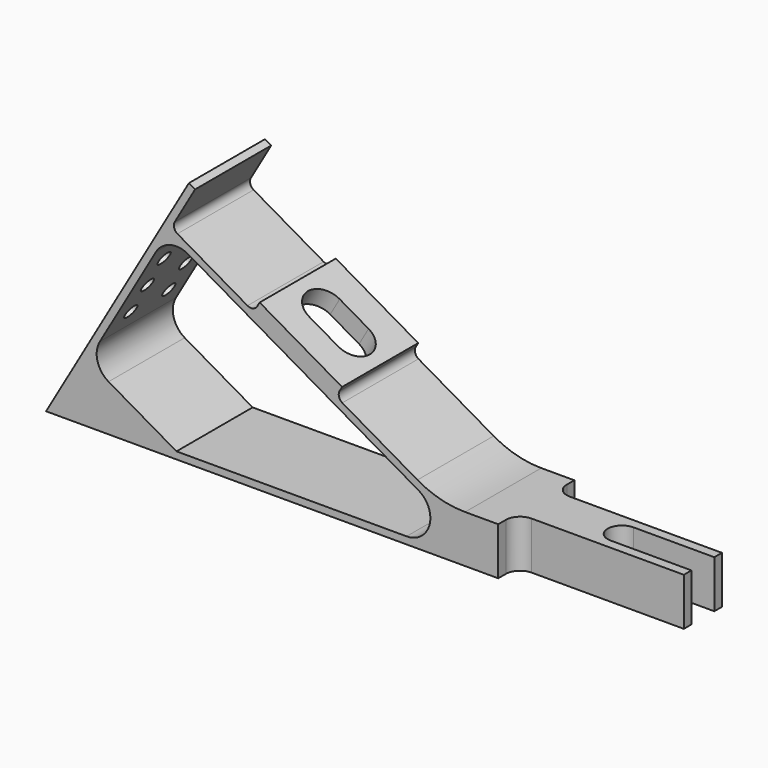
from build123d import *

# Parameters (mm, degrees)
F1_DEPTH      = 10
F3_DEPTH      = 20.001
F3_DEPTH_BACK = 197
F4_R          = 1.5
F5_DEPTH      = 1.5
F4_R_2        = 4.25
F6_DEPTH      = 112.584302492
F4_R_3        = 5.5
F7_DEPTH      = 2
F8_W          = 17
F8_H          = 6
F9_DEPTH      = 10.001
F10_W         = 7
F10_H         = 8
F11_DEPTH     = 4


# Not quite as in the source:
# - an extrude ends at something that could not be found from the text; its depth is read off the source's solid


with BuildPart() as f1:
    # F0 (on Front) → F1 (new body, symmetric)
    with BuildSketch(Plane.XZ):
        with BuildLine():
            Line((30, 51.9615242271), (0, 0))
            Line((0, 0), (130, 0))
            Line((130, 0), (130, 10))
            Line((130, 10), (88.0384757729, 10))
            ThreePointArc((88.0384757729, 10), (82.8620948709, 10.6814834742), (78.0384757729, 12.6794919243))
            Line((78.0384757729, 12.6794919243), (62.2390923627, 21.8012701892))
            ThreePointArc((62.2390923627, 21.8012701892), (61.5402036233, 22.7120797272), (61.6900542571, 23.8503082949))
            Line((61.6900542571, 23.8503082949), (62.1900542571, 24.7163336987))
            Line((62.1900542571, 24.7163336987), (44.8695461814, 34.7163336987))
            Line((44.8695461814, 34.7163336987), (44.3695461814, 33.8503082949))
            ThreePointArc((44.3695461814, 33.8503082949), (43.4587366433, 33.1514195555), (42.3205080757, 33.3012701892))
            Line((42.3205080757, 33.3012701892), (27.5980762114, 41.8012701892))
            ThreePointArc((27.5980762114, 41.8012701892), (26.8991874719, 42.7120797272), (27.0490381057, 43.8503082949))
            Line((27.0490381057, 43.8503082949), (31.2990381057, 51.2115242271))
            Line((31.2990381057, 51.2115242271), (30, 51.9615242271))
        make_face()
        with BuildLine():
            ThreePointArc((23.0490381057, 36.9221050646), (26.0850698991, 39.2517341961), (29.8791651246, 38.7522320835))
            Line((29.8791651246, 38.7522320835), (78.2416697508, 10.8301270189))
            ThreePointArc((78.2416697508, 10.8301270189), (80.5712988822, 5.2059047745), (75.7416697508, 1.5))
            Line((75.7416697508, 1.5), (27.4019237886, 1.5))
            Line((27.4019237886, 1.5), (13.1291651246, 9.7403810568))
            ThreePointArc((13.1291651246, 9.7403810568), (10.7995359932, 12.7764128502), (11.2990381057, 16.5705080757))
            Line((11.2990381057, 16.5705080757), (23.0490381057, 36.9221050646))
        make_face(mode=Mode.SUBTRACT)
        with BuildLine():
            Line((78.2416697508, 10.8301270189), (29.8791651246, 38.7522320835))
            ThreePointArc((29.8791651246, 38.7522320835), (26.0850698991, 39.2517341961), (23.0490381057, 36.9221050646))
            Line((23.0490381057, 36.9221050646), (11.2990381057, 16.5705080757))
            ThreePointArc((11.2990381057, 16.5705080757), (10.7995359932, 12.7764128502), (13.1291651246, 9.7403810568))
            Line((13.1291651246, 9.7403810568), (27.4019237886, 1.5))
            Line((27.4019237886, 1.5), (75.7416697508, 1.5))
            ThreePointArc((75.7416697508, 1.5), (80.5712988822, 5.2059047745), (78.2416697508, 10.8301270189))
        make_face()
    extrude(amount=F1_DEPTH, both=True)

    # F2 (on face) → F3 (cut, two sides)
    with BuildSketch(Plane.XZ.offset(10)) as f3_sk:
        with BuildLine():
            ThreePointArc((29.8791651246, 38.7522320835), (26.0850698991, 39.2517341961), (23.0490381057, 36.9221050646))
            Line((23.0490381057, 36.9221050646), (11.2990381057, 16.5705080757))
            ThreePointArc((11.2990381057, 16.5705080757), (10.7995359932, 12.7764128502), (13.1291651246, 9.7403810568))
            Line((13.1291651246, 9.7403810568), (27.4019237886, 1.5))
            Line((27.4019237886, 1.5), (75.7416697508, 1.5))
            ThreePointArc((75.7416697508, 1.5), (80.5712988822, 5.2059047745), (78.2416697508, 10.8301270189))
            Line((78.2416697508, 10.8301270189), (29.8791651246, 38.7522320835))
        make_face()
    extrude(amount=-F3_DEPTH, mode=Mode.SUBTRACT)
    extrude(f3_sk.sketch, amount=F3_DEPTH_BACK, mode=Mode.SUBTRACT)

    # F4 (on face) → F5 (cut, through all)
    with BuildSketch(Plane(origin=(0, 0, 0), x_dir=(0, -1, 0), z_dir=(-0.8660254038, 0, 0.5))):
        with Locations((-5, 25)):
            Circle(F4_R)
        with Locations((-5, 32)):
            Circle(F4_R)
        with Locations((-5, 39)):
            Circle(F4_R)
        with Locations((5, 39)):
            Circle(F4_R)
        with Locations((5, 32)):
            Circle(F4_R)
        with Locations((5, 25)):
            Circle(F4_R)
    extrude(amount=-F5_DEPTH, mode=Mode.SUBTRACT)

    # F4 (on face) → F6 (cut, through all)
    with BuildSketch(Plane(origin=(0, 0, 0), x_dir=(0, -1, 0), z_dir=(-0.8660254038, 0, 0.5))):
        with Locations((0, 10)):
            Circle(F4_R_2)
    extrude(amount=-F6_DEPTH, mode=Mode.SUBTRACT)

    # F4 (on face) → F7 (cut)
    with BuildSketch(Plane(origin=(0, 0, 0), x_dir=(0, -1, 0), z_dir=(-0.8660254038, 0, 0.5))):
        with Locations((0, 10)):
            Circle(F4_R_3)
        with Locations((0, 10)):
            Circle(F4_R_2, mode=Mode.SUBTRACT)
    extrude(amount=-F7_DEPTH, mode=Mode.SUBTRACT)

    # F8 (on face) → F9 (cut, through all)
    with BuildSketch(Plane.XY.offset(10)):
        with Locations((121.5, 0)):
            Rectangle(F8_W, F8_H)
        with BuildLine():
            ThreePointArc((113, 3), (110, 0), (113, -3))
            Line((113, -3), (113, 3))
        make_face()
        with BuildLine():
            Line((130, -10), (130, -5))
            Line((130, -5), (98, -5))
            ThreePointArc((98, -5), (95.8786796564, -5.8786796564), (95, -8))
            Line((95, -8), (95, -10))
            Line((95, -10), (130, -10))
        make_face()
        with BuildLine():
            Line((98, 5), (130, 5))
            Line((130, 5), (130, 10))
            Line((130, 10), (95, 10))
            Line((95, 10), (95, 8))
            ThreePointArc((95, 8), (95.8786796564, 5.8786796564), (98, 5))
        make_face()
    extrude(amount=-F9_DEPTH, mode=Mode.SUBTRACT)

    # F10 (on face) → F11 (cut, through all)
    with BuildSketch(Plane(origin=(26.25, 0, 45.4663336987), x_dir=(0.8660254038, 0, -0.5), z_dir=(0.5, 0, 0.8660254038))):
        with BuildLine():
            ThreePointArc((28, 4), (24, 0), (28, -4))
            Line((28, -4), (28, 4))
        make_face()
        with Locations((31.5, 0)):
            Rectangle(F10_W, F10_H)
        with BuildLine():
            Line((35, 4), (35, -4))
            ThreePointArc((35, -4), (39, 0), (35, 4))
        make_face()
    extrude(amount=-F11_DEPTH, mode=Mode.SUBTRACT)


solid = f1.part
